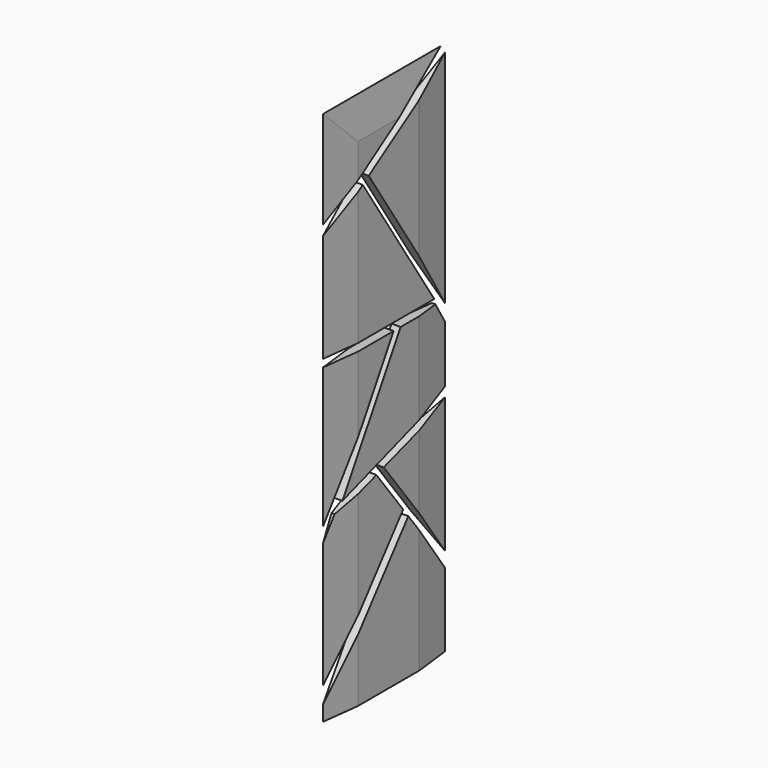
from build123d import *

# Parameters (mm, degrees)
F1_DEPTH    = 0.762
F2_SIZE2    = 0.762
F2_SIZE     = 6.35
F2_2_SIZE2  = 0.76199
F2_2_SIZE   = 6.34999
F2_3_SIZE2  = 0.762
F2_3_SIZE   = 6.35
F2_4_SIZE2  = 0.76199
F2_4_SIZE   = 6.34999
F2_5_SIZE2  = 0.762
F2_5_SIZE   = 6.35
F2_6_SIZE2  = 0.76199
F2_6_SIZE   = 6.34999
F2_7_SIZE2  = 0.762
F2_7_SIZE   = 6.35
F2_8_SIZE2  = 0.76199
F2_8_SIZE   = 6.34999
F2_9_SIZE2  = 0.762
F2_9_SIZE   = 6.35
F2_10_SIZE2 = 0.76199
F2_10_SIZE  = 6.34999
F2_11_SIZE2 = 0.762
F2_11_SIZE  = 6.35
F2_12_SIZE2 = 0.76199
F2_12_SIZE  = 6.34999
F2_13_SIZE2 = 0.762
F2_13_SIZE  = 6.35
F2_14_SIZE2 = 0.76199
F2_14_SIZE  = 6.34999
F2_15_SIZE2 = 0.762
F2_15_SIZE  = 6.35
F2_16_SIZE2 = 0.76199
F2_16_SIZE  = 6.34999
F3_SIZE2    = 6.34999
F3_SIZE     = 0.76199


# Not quite as in the source:
# - a fillet or chamfer is up to 0.001 mm smaller than in the source, because OpenCascade refuses the exact size


with BuildPart() as f1:
    # F0 (on Right) → F1 (new body, symmetric)
    with BuildSketch(Plane.YZ):
        Polygon((-12.7, 51.828302443), (-12.7, 28.5059732678), (1.0529800206, 51.828302443), align=None)
    extrude(amount=F1_DEPTH, both=True)

    # F2#13
    f2_13_edges = [f1.edges().sort_by_distance(p)[0] for p in [
        (-0.762, -12.7, 40.167138),
    ]]
    f2_13_side = f1.faces().sort_by_distance((-0.762, -8.115673, 44.054193))[0]
    chamfer(f2_13_edges, length=F2_13_SIZE, length2=F2_13_SIZE2, reference=f2_13_side)

    # F2#14 (size 6.35 and 0.762 in the source; OpenCascade refuses exactly that, so slightly less here)
    f2_14_edges = [f1.edges().sort_by_distance(p)[0] for p in [
        (0.762, -12.7, 40.167138),
    ]]
    f2_14_side = f1.faces().sort_by_distance((0.762, -8.115673, 44.054193))[0]
    chamfer(f2_14_edges, length=F2_14_SIZE, length2=F2_14_SIZE2, reference=f2_14_side)


with BuildPart() as f1b:
    # F0 (on Right) → F1, piece 2 (new body, symmetric)
    with BuildSketch(Plane.YZ):
        Polygon((-12.7, 26.0336679026), (-12.7, 5.2599026822), (3.0286672094, 24.9264711231), (-2.5214019575, 32.2336712183), (-10.594333522, 29.6044610441), align=None)
    extrude(amount=F1_DEPTH, both=True)

    # F2#15
    f2_15_edges = [f1b.edges().sort_by_distance(p)[0] for p in [
        (-0.762, -12.7, 15.646785),
    ]]
    f2_15_side = f1b.faces().sort_by_distance((-0.762, -6.710937, 21.407423))[0]
    chamfer(f2_15_edges, length=F2_15_SIZE, length2=F2_15_SIZE2, reference=f2_15_side)

    # F2#16 (size 6.35 and 0.762 in the source; OpenCascade refuses exactly that, so slightly less here)
    f2_16_edges = [f1b.edges().sort_by_distance(p)[0] for p in [
        (0.762, -12.7, 15.646785),
    ]]
    f2_16_side = f1b.faces().sort_by_distance((0.762, -6.710937, 21.407423))[0]
    chamfer(f2_16_edges, length=F2_16_SIZE, length2=F2_16_SIZE2, reference=f2_16_side)


with BuildPart() as f1c:
    # F0 (on Right) → F1, piece 3 (new body, symmetric)
    with BuildSketch(Plane.YZ):
        Polygon((-4.1242268054, 76.6329197301), (12.7, 50.884090213), (12.7, 87.6258313656), align=None)
    extrude(amount=F1_DEPTH, both=True)

    # F2#3
    f2_3_edges = [f1c.edges().sort_by_distance(p)[0] for p in [
        (0.762, 12.7, 69.254961),
    ]]
    f2_3_side = f1c.faces().sort_by_distance((0.762, 7.091924, 71.71428))[0]
    chamfer(f2_3_edges, length=F2_3_SIZE, length2=F2_3_SIZE2, reference=f2_3_side)

    # F2#4 (size 6.35 and 0.762 in the source; OpenCascade refuses exactly that, so slightly less here)
    f2_4_edges = [f1c.edges().sort_by_distance(p)[0] for p in [
        (-0.762, 12.7, 69.254961),
    ]]
    f2_4_side = f1c.faces().sort_by_distance((-0.762, 7.091924, 71.71428))[0]
    chamfer(f2_4_edges, length=F2_4_SIZE, length2=F2_4_SIZE2, reference=f2_4_side)


with BuildPart() as f1d:
    # F0 (on Right) → F1, piece 4 (new body, symmetric)
    with BuildSketch(Plane.YZ):
        Polygon((-9.5868147053, 31.313013333), (12.7, 38.7808382511), (12.7, 48.1682026787), (10.3084991155, 51.828302443), (2.510877559, 51.828302443), align=None)
    extrude(amount=F1_DEPTH, both=True)

    # F2
    f2_edges = [f1d.edges().sort_by_distance(p)[0] for p in [
        (0.762, 12.7, 43.47452),
    ]]
    f2_side = f1d.faces().sort_by_distance((0.762, 3.707113, 42.31436))[0]
    chamfer(f2_edges, length=F2_SIZE, length2=F2_SIZE2, reference=f2_side)

    # F2#2 (size 6.35 and 0.762 in the source; OpenCascade refuses exactly that, so slightly less here)
    f2_2_edges = [f1d.edges().sort_by_distance(p)[0] for p in [
        (-0.762, 12.7, 43.47452),
    ]]
    f2_2_side = f1d.faces().sort_by_distance((-0.762, 3.707113, 42.31436))[0]
    chamfer(f2_2_edges, length=F2_2_SIZE, length2=F2_2_SIZE2, reference=f2_2_side)


with BuildPart() as f1e:
    # F0 (on Right) → F1, piece 5 (new body, symmetric)
    with BuildSketch(Plane.YZ):
        Polygon((-1.0126563937, 32.7250428043), (12.7, 14.6710112068), (12.7, 37.1910110116), align=None)
    extrude(amount=F1_DEPTH, both=True)

    # F2#5
    f2_5_edges = [f1e.edges().sort_by_distance(p)[0] for p in [
        (0.762, 12.7, 25.931011),
    ]]
    f2_5_side = f1e.faces().sort_by_distance((0.762, 8.129115, 28.195688))[0]
    chamfer(f2_5_edges, length=F2_5_SIZE, length2=F2_5_SIZE2, reference=f2_5_side)

    # F2#6 (size 6.35 and 0.762 in the source; OpenCascade refuses exactly that, so slightly less here)
    f2_6_edges = [f1e.edges().sort_by_distance(p)[0] for p in [
        (-0.762, 12.7, 25.931011),
    ]]
    f2_6_side = f1e.faces().sort_by_distance((-0.762, 8.129115, 28.195688))[0]
    chamfer(f2_6_edges, length=F2_6_SIZE, length2=F2_6_SIZE2, reference=f2_6_side)


with BuildPart() as f1f:
    # F0 (on Right) → F1, piece 6 (new body, symmetric)
    with BuildSketch(Plane.YZ):
        Polygon((-12.7, 0), (0, 0), (12.7, 0), (12.7, 12.1932309121), (4.1025487481, 23.5126027467), (-12.7, 2.5032908618), align=None)
    extrude(amount=F1_DEPTH, both=True)

    # F2#7
    f2_7_edges = [f1f.edges().sort_by_distance(p)[0] for p in [
        (0.762, 12.7, 6.096615),
        (0.762, -12.7, 1.251645),
    ]]
    f2_7_side = f1f.faces().sort_by_distance((0.762, 2.081715, 8.457296))[0]
    chamfer(f2_7_edges, length=F2_7_SIZE, length2=F2_7_SIZE2, reference=f2_7_side)

    # F2#8 (size 6.35 and 0.762 in the source; OpenCascade refuses exactly that, so slightly less here)
    f2_8_edges = [f1f.edges().sort_by_distance(p)[0] for p in [
        (-0.762, -12.7, 1.251645),
        (-0.762, 12.7, 6.096615),
    ]]
    f2_8_side = f1f.faces().sort_by_distance((-0.762, 2.081715, 8.457296))[0]
    chamfer(f2_8_edges, length=F2_8_SIZE, length2=F2_8_SIZE2, reference=f2_8_side)


with BuildPart() as f1g:
    # F0 (on Right) → F1, piece 7 (new body, symmetric)
    with BuildSketch(Plane.YZ):
        Polygon((11.7632681504, 88.9), (-12.7, 88.9), (-12.7, 72.6716294885), align=None)
    extrude(amount=F1_DEPTH, both=True)

    # F2#9
    f2_9_edges = [f1g.edges().sort_by_distance(p)[0] for p in [
        (-0.762, -12.7, 80.785815),
        (-0.762, -0.468366, 88.9),
    ]]
    f2_9_side = f1g.faces().sort_by_distance((-0.762, -4.545577, 83.490543))[0]
    chamfer(f2_9_edges, length=F2_9_SIZE, length2=F2_9_SIZE2, reference=f2_9_side)

    # F2#10 (size 6.35 and 0.762 in the source; OpenCascade refuses exactly that, so slightly less here)
    f2_10_edges = [f1g.edges().sort_by_distance(p)[0] for p in [
        (0.762, -12.7, 80.785815),
    ]]
    f2_10_side = f1g.faces().sort_by_distance((0.762, -4.545577, 83.490543))[0]
    chamfer(f2_10_edges, length=F2_10_SIZE, length2=F2_10_SIZE2, reference=f2_10_side)

    # F3 (size 0.762 and 6.35 in the source; OpenCascade refuses exactly that, so slightly less here)
    f3_edges = [f1g.edges().sort_by_distance(p)[0] for p in [
        (0.762, 2.706629, 88.9),
    ]]
    f3_side = f1g.faces().sort_by_distance((0.362059, 1.040187, 88.9))[0]
    chamfer(f3_edges, length=F3_SIZE, length2=F3_SIZE2, reference=f3_side)


with BuildPart() as f1h:
    # F0 (on Right) → F1, piece 8 (new body, symmetric)
    with BuildSketch(Plane.YZ):
        Polygon((-5.3678452737, 75.8203422436), (-12.7, 71.0295289755), (-12.7, 53.0840971504), (9.487965702, 53.0840971504), align=None)
    extrude(amount=F1_DEPTH, both=True)

    # F2#11
    f2_11_edges = [f1h.edges().sort_by_distance(p)[0] for p in [
        (-0.762, -12.7, 62.056813),
    ]]
    f2_11_side = f1h.faces().sort_by_distance((-0.762, -4.389957, 61.900294))[0]
    chamfer(f2_11_edges, length=F2_11_SIZE, length2=F2_11_SIZE2, reference=f2_11_side)

    # F2#12 (size 6.35 and 0.762 in the source; OpenCascade refuses exactly that, so slightly less here)
    f2_12_edges = [f1h.edges().sort_by_distance(p)[0] for p in [
        (0.762, -12.7, 62.056813),
    ]]
    f2_12_side = f1h.faces().sort_by_distance((0.762, -4.389957, 61.900294))[0]
    chamfer(f2_12_edges, length=F2_12_SIZE, length2=F2_12_SIZE2, reference=f2_12_side)


solid = Compound([f1.part, f1b.part, f1c.part, f1d.part, f1e.part, f1f.part, f1g.part, f1h.part])
